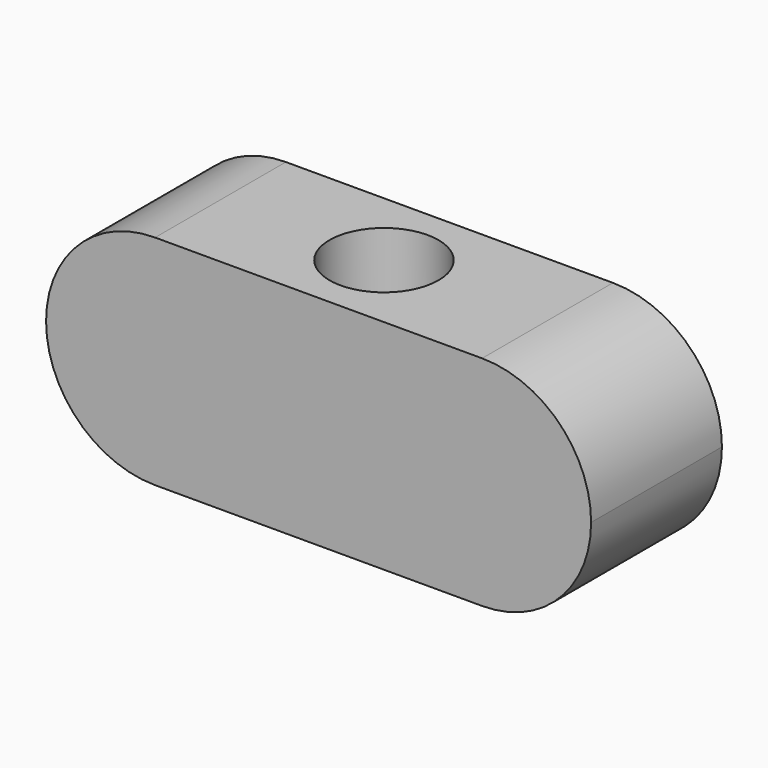
from build123d import *

# Parameters (mm, degrees)
F0_W     = 127
F0_H     = 50.8
F1_DEPTH = 38.1
F2_R     = 25.39999
F3_R     = 12.2082879552
F3_R_2   = 12.7
F4_DEPTH = 19.05
F5_R     = 12.7
F6_DEPTH = 50.8


# Not quite as in the source:
# - a fillet or chamfer is up to 0.001 mm smaller than in the source, because OpenCascade refuses the exact size


with BuildPart() as f1:
    # F0 (on Front) → F1 (new body)
    with BuildSketch(Plane.XZ):
        Rectangle(F0_W, F0_H)
    extrude(amount=F1_DEPTH)

    # F2 (radius 25.4 in the source; OpenCascade refuses exactly that, so slightly less here)
    f2_edges = [f1.edges().sort_by_distance(p)[0] for p in [
        (63.5, -19.05, 25.4),
        (63.5, -19.05, -25.4),
        (-63.5, -19.05, 25.4),
        (-63.5, -19.05, -25.4),
    ]]
    fillet(f2_edges, radius=F2_R)

    # F3 (on face) → F4 (cut)
    with BuildSketch(Plane(origin=(0, 0, 0), x_dir=(-1, 0, 0), z_dir=(0, 1, 0))):
        with Locations((47.625, 0)):
            Circle(F3_R)
        with Locations((-47.625, 0)):
            Circle(F3_R_2)
    extrude(amount=-F4_DEPTH, mode=Mode.SUBTRACT)

    # F5 (on face) → F6 (cut)
    with BuildSketch(Plane.XY.offset(25.4)):
        with Locations((0, -19.05)):
            Circle(F5_R)
    extrude(amount=-F6_DEPTH, mode=Mode.SUBTRACT)


solid = f1.part
